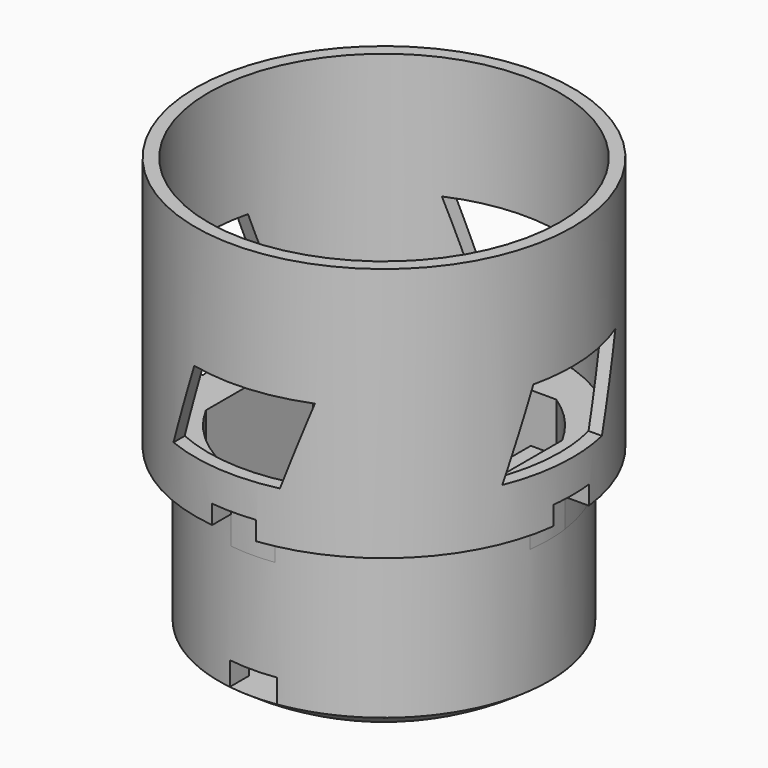
from build123d import *
from build123d import SkipClean  # not in build123d's __all__

# Parameters (mm, degrees)
F0_R      = 35
F0_R_2    = 30
F1_DEPTH  = 10
F2_W      = 9.35
F2_H      = 20
F3_DEPTH  = 10
F5_R      = 35
F5_R_2    = 30
F6_DEPTH  = 26.4
F8_COUNT  = 4
F11_W     = 33
F11_H     = 4.9450603673
F14_DEPTH = 37
F15_W     = 5.4
F15_H     = 16
F15_H_2   = 7
F16_DEPTH = 12
F17_W     = 5.0788592132
F17_H     = 28.4684949474
F18_DEPTH = 36
F19_W     = 10
F19_H     = 5
F20_DEPTH = 54.2
F21_R     = 40
F21_R_2   = 37.25
F22_DEPTH = 50
F23_R     = 40
F23_R_2   = 34.3880448287
F24_DEPTH = 4
F30_DEPTH = 20.7
F32_DEPTH = 25
F34_DEPTH = 25
F36_DEPTH = 25
F38_DEPTH = 10


# Not quite as in the source:
# - a feature names something its author has since deleted; it is built from what else it names


with BuildPart() as f1:
    # F0 (on Top) → F1 (new body)
    with BuildSketch(Plane.XY):
        Circle(F0_R)
        Circle(F0_R_2, mode=Mode.SUBTRACT)
    extrude(amount=-F1_DEPTH)

    # F2 (on Top) → F3 (join)
    with BuildSketch(Plane.XY):
        with Locations((0, 44)):
            Rectangle(F2_W, F2_H)
    extrude(amount=-F3_DEPTH)

    # F5 (on face) → F6 (join)
    with BuildSketch(Plane(origin=(0, 0, -10), x_dir=(1, 0, 0), z_dir=(0, 0, -1))):
        Circle(F5_R)
        Circle(F5_R_2, mode=Mode.SUBTRACT)
    extrude(amount=F6_DEPTH)


with BuildPart() as f8_1:
    # F8: instance of F1
    add(f1.part.rotate(Axis((0, 0, 27.0554148592), (0, 0, -1)), 1 * 360 / F8_COUNT), clean=False)


with BuildPart() as f8_2:
    # F8: instance of F1
    add(f1.part.rotate(Axis((0, 0, 27.0554148592), (0, 0, -1)), 2 * 360 / F8_COUNT), clean=False)


with BuildPart() as f8_3:
    # F8: instance of F1
    add(f1.part.rotate(Axis((0, 0, 27.0554148592), (0, 0, -1)), 3 * 360 / F8_COUNT), clean=False)


with BuildPart() as f1_1:
    add(f1.part, clean=False)

    add(f8_1.part)  # F10 merges F8_1

    add(f8_2.part)  # F10 merges F8_2

    add(f8_3.part)  # F10 merges F8_3
    # F9 (on Right) → F10 (revolve)
    with BuildSketch(Plane.YZ):
        with BuildLine():
            Line((0, -48.0663776398), (0, -36.3997630775))
            Line((0, -36.3997630775), (-34.9988900125, -36.3997630775))
            ThreePointArc((-34.9988900125, -36.3997630775), (-18.4183780329, -44.9897943213), (0, -48.0663776398))
        make_face()
    revolve(axis=Axis((0, 0, 27.0554148592), (0, 0, -1)))

    # F12: union 

    # F13: union 

    # F11 (on Top) → F14 (join)
    with BuildSketch(Plane.XY):
        with Locations((0, 27.5274698164)):
            Rectangle(F11_W, F11_H)
    extrude(amount=-F14_DEPTH)

    # F15 (on face) → F16 (join)
    with BuildSketch(Plane.XZ.offset(-25.0549396327)):
        Polygon((-16.5000000774, -26.3998815387), (-16.5000000774, -36.3998815387), (16.5, -36.3998815387), (16.5, -26.3998815387), (-11.1000000774, -26.3998815387), align=None)
        with Locations((-13.8000000774, -18.3998815387)):
            Rectangle(F15_W, F15_H)
        with Locations((13.8, -13.8998815387)):
            Rectangle(F15_W, F15_H_2)
    extrude(amount=F16_DEPTH)

    # F17 (on face) → F18 (join)
    with BuildSketch(Plane.XY):
        with Locations((-28.947500321, 0)):
            Rectangle(F17_W, F17_H)
        with Locations((28.947500321, 0)):
            Rectangle(F17_W, F17_H)
    extrude(amount=-F18_DEPTH)

    # F19 (on face) → F20 (cut)
    with BuildSketch(Plane.XZ.offset(-13.0549396327)):
        with Locations((0, -33.8997630775)):
            Rectangle(F19_W, F19_H)
    extrude(amount=F20_DEPTH, mode=Mode.SUBTRACT)

    # F21 (on face) → F22 (join)
    with BuildSketch(Plane.XY):
        Circle(F21_R)
        Circle(F21_R_2, mode=Mode.SUBTRACT)
    extrude(amount=F22_DEPTH)

    # F23 (on face) → F24 (join)
    with BuildSketch(Plane.XY):
        Circle(F23_R)
        Circle(F23_R_2, mode=Mode.SUBTRACT)
    extrude(amount=-F24_DEPTH)

    # F29 (on offset) → F30 (cut)
    with BuildSketch(Plane.XZ.offset(44)):
        Polygon((9.0839202169, 7), (15, 24), (-9.0839202169, 24), (-15, 7), align=None)
    extrude(amount=-F30_DEPTH, mode=Mode.SUBTRACT)

    # F31 (on offset) → F32 (cut)
    with BuildSketch(Plane.XZ.offset(-44)):
        Polygon((9.0839202169, 24), (-15, 24), (-9.0839202169, 7), (15, 7), align=None)
    extrude(amount=F32_DEPTH, mode=Mode.SUBTRACT)

    # F33 (on offset) → F34 (cut)
    with BuildSketch(Plane.YZ.offset(44)):
        Polygon((9.0839202169, 7), (15, 24), (-9.0839202169, 24), (-15, 7), align=None)
    extrude(amount=-F34_DEPTH, mode=Mode.SUBTRACT)

    # F35 (on offset) → F36 (cut)
    with BuildSketch(Plane.YZ.offset(-44)):
        Polygon((9.0839202169, 24), (-15, 24), (-9.0839202169, 7), (15, 7), align=None)
    extrude(amount=F36_DEPTH, mode=Mode.SUBTRACT)

    # F37 (on face) → F38 (cut)
    with BuildSketch(Plane(origin=(0, 0, -10), x_dir=(1, 0, 0), z_dir=(0, 0, -1))):
        with BuildLine():
            ThreePointArc((4.675, -34.6863716033), (0, -35), (-4.675, -34.6863716033))
            Line((-4.675, -34.6863716033), (-4.675, -54))
            Line((-4.675, -54), (4.675, -54))
            Line((4.675, -54), (4.675, -34.6863716033))
        make_face()
        with BuildLine():
            Line((54, -4.675), (54, 4.675))
            Line((54, 4.675), (34.6863716033, 4.675))
            ThreePointArc((34.6863716033, 4.675), (35, 0), (34.6863716033, -4.675))
            Line((34.6863716033, -4.675), (54, -4.675))
        make_face()
        with BuildLine():
            Line((4.675, 54), (-4.675, 54))
            Line((-4.675, 54), (-4.675, 34.6863716033))
            ThreePointArc((-4.675, 34.6863716033), (0, 35), (4.675, 34.6863716033))
            Line((4.675, 34.6863716033), (4.675, 54))
        make_face()
        with BuildLine():
            Line((-54, 4.675), (-54, -4.675))
            Line((-54, -4.675), (-34.6863716033, -4.675))
            ThreePointArc((-34.6863716033, -4.675), (-35, 0), (-34.6863716033, 4.675))
            Line((-34.6863716033, 4.675), (-54, 4.675))
        make_face()
    with SkipClean():  # cleaning this boolean's faces spoils the solid; the shape is the same uncleaned
        extrude(amount=-F38_DEPTH, mode=Mode.SUBTRACT)


solid = f1_1.part
